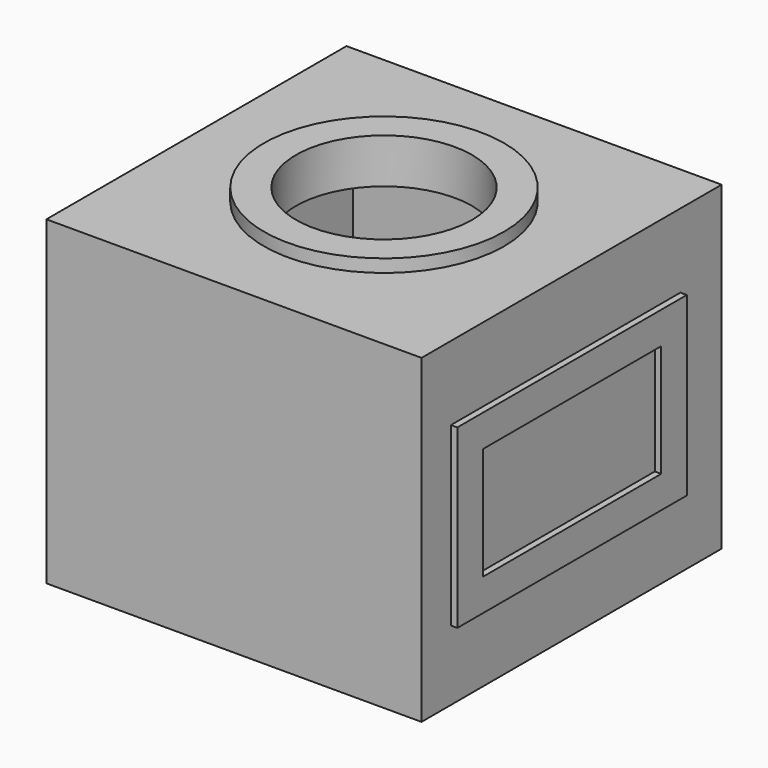
from build123d import *

# Parameters (mm, degrees)
F0_W          = 29.7304940177
F0_H          = 29.7304925771
F1_DEPTH      = 25.4
F2_R          = 9.516573444
F3_DEPTH      = 1.016
F4_T          = -2.54
F5_W          = 22.7350834757
F5_H          = 13.9908185229
F6_DEPTH      = 0.508
F7_T          = 2.54
F7_T3_DEPTH   = 25.4
F7_T5_DEPTH   = 29.7304925771
F7_T7_DEPTH   = 29.7304940177
F7_T9_DEPTH   = 27.8150834757
F7_T11_DEPTH  = 19.0708185229
F9_DEPTH      = 1.27
F10_T         = 2.54
F10_T3_DEPTH  = 25.4
F10_T5_DEPTH  = 29.7304925771
F10_T7_DEPTH  = 29.7304940177
F10_T9_DEPTH  = 20.819671886
F10_T11_DEPTH = 19.0130124822
F10_T13_DEPTH = 18.3381282199
F10_T15_DEPTH = 27.8150834757
F10_T17_DEPTH = 19.0708185229
F10_T19_DEPTH = 22.7350834757
F10_T21_DEPTH = 5.588
F10_T23_DEPTH = 13.9908185229
F12_DEPTH     = 1.016
F14_DEPTH     = 0.762


# Not quite as in the source:
# - a shell that OpenCascade refuses in one call is made with other operations: the cavity is built on its own and cut out


with BuildPart() as f1:
    # F0 (on Top) → F1 (new body)
    with BuildSketch(Plane.XY):
        with Locations((15.1567222201, 15.010983996)):
            Rectangle(F0_W, F0_H)
    extrude(amount=F1_DEPTH)

    # F2 (on face) → F3 (join)
    with BuildSketch(Plane.XY.offset(25.4)):
        with Locations((15.1567222201, 15.010983996)):
            Circle(F2_R)
    extrude(amount=F3_DEPTH)

    # F4
    f4_openings = [f1.faces().sort_by_distance(p)[0] for p in [
        (15.156722, 15.010984, 26.416),
    ]]
    offset(amount=F4_T, openings=f4_openings, kind=Kind.INTERSECTION)

    # F5 (on face) → F6 (join)
    with BuildSketch(Plane.YZ.offset(30.021969229)):
        with Locations((14.4280334935, 12.5334435143)):
            Rectangle(F5_W, F5_H)
    extrude(amount=F6_DEPTH)

    # F7: shell of thickness 2.54, made by hand


with BuildPart() as f7_core1:
    # F7_t2: copy of F1
    add(f1.part)

    # the walls: a layer under each face that stays
    f7_faces = [f7_core1.faces().sort_by_distance(p)[0] for p in [
        (2.8314752113, 15.010983996, 12.7),
        (15.1567222201, 27.3362302846, 12.7),
        (6.9398908809, 6.794153137, 22.86),
        (15.1567222201, 2.6857377075, 12.7),
        (15.1567222201, 15.010983996, 2.54),
        (27.481969229, 15.010983996, 12.7),
        (8.1801487762, 15.010983996, 24.638),
        (8.8123399241, 8.6666017001, 26.416),
        (5.6401487762, 15.010983996, 25.908),
        (5.2465575476, 5.1008198037, 25.4),
        (0.2914752113, 15.010983996, 12.7),
        (15.1567222201, 29.8762302846, 12.7),
        (15.1567222201, 0.1457377075, 12.7),
        (30.021969229, 5.1008198037, 21.1666666667),
        (15.1567222201, 15.010983996, 0),
        (30.275969229, 14.4280334935, 5.5380342528),
        (30.275969229, 3.0604917556, 12.5334435143),
        (30.275969229, 14.4280334935, 19.5288527757),
        (30.275969229, 25.7955752313, 12.5334435143),
    ]]
    thicken(f7_faces, amount=-F7_T, mode=Mode.SUBTRACT)

    # F7_s4 → F7_t3 (cut)
    with BuildSketch(Plane.XY):
        Polygon((2.8568752113, 27.3108302846), (0.2914752113, 27.3362302846), (0.2914752113, 29.8762302846), (2.8314752113, 29.8762302846), align=None)
        Polygon((2.8568752113, 2.7111377075), (0.2914752113, 2.6857377075), (0.2914752113, 0.1457377075), (2.8314752113, 0.1457377075), align=None)
        Polygon((27.456569229, 27.3108302846), (27.481969229, 29.8762302846), (30.021969229, 29.8762302846), (30.021969229, 27.3362302846), align=None)
        Polygon((27.456569229, 2.7111377075), (27.481969229, 0.1457377075), (30.021969229, 0.1457377075), (30.021969229, 2.6857377075), align=None)
    extrude(amount=F7_T3_DEPTH, mode=Mode.SUBTRACT)

    # F7_s6 → F7_t5 (cut)
    with BuildSketch(Plane.XZ.offset(-29.8762302846)):
        Polygon((2.8568752113, 22.8346), (0.2914752113, 22.86), (0.2914752113, 25.4), (2.8314752113, 25.4), align=None)
        Polygon((2.8568752113, 2.5654), (0.2914752113, 2.54), (0.2914752113, 0), (2.8314752113, 0), align=None)
        Polygon((27.456569229, 22.8346), (27.481969229, 25.4), (30.021969229, 25.4), (30.021969229, 22.86), align=None)
        Polygon((27.456569229, 2.5654), (27.481969229, 0), (30.021969229, 0), (30.021969229, 2.54), align=None)
    extrude(amount=F7_T5_DEPTH, mode=Mode.SUBTRACT)

    # F7_s8 → F7_t7 (cut)
    with BuildSketch(Plane.YZ.offset(0.2914752113)):
        Polygon((27.3108302846, 22.8346), (29.8762302846, 22.86), (29.8762302846, 25.4), (27.3362302846, 25.4), align=None)
        Polygon((27.3108302846, 2.5654), (29.8762302846, 2.54), (29.8762302846, 0), (27.3362302846, 0), align=None)
        Polygon((2.7111377075, 22.8346), (2.6857377075, 25.4), (0.1457377075, 25.4), (0.1457377075, 22.86), align=None)
        Polygon((2.7111377075, 2.5654), (0.1457377075, 2.54), (0.1457377075, 0), (2.6857377075, 0), align=None)
    extrude(amount=F7_T7_DEPTH, mode=Mode.SUBTRACT)

    # F7_s10 → F7_t9 (cut)
    with BuildSketch(Plane.XZ.offset(-28.3355752313)):
        Polygon((30.047369229, 5.5126342528), (27.481969229, 5.5380342528), (27.481969229, 8.0780342528), (30.021969229, 8.0780342528), align=None)
        Polygon((30.047369229, 19.5542527757), (27.481969229, 19.5288527757), (27.481969229, 16.9888527757), (30.021969229, 16.9888527757), align=None)
    extrude(amount=F7_T9_DEPTH, mode=Mode.SUBTRACT)

    # F7_s12 → F7_t11 (cut)
    with BuildSketch(Plane.XY.offset(2.9980342528)):
        Polygon((30.047369229, 3.0350917556), (27.481969229, 3.0604917556), (27.481969229, 5.6004917556), (30.021969229, 5.6004917556), align=None)
        Polygon((30.047369229, 25.8209752313), (27.481969229, 25.7955752313), (27.481969229, 23.2555752313), (30.021969229, 23.2555752313), align=None)
    extrude(amount=F7_T11_DEPTH, mode=Mode.SUBTRACT)

    # F7_s13 → F7_t14 (revolve, cut)
    with BuildSketch(Plane.XZ.offset(-15.010983996)):
        Polygon((24.6986956641, 25.4254), (22.1332956641, 25.4), (22.1332956641, 22.86), (24.6732956641, 22.86), align=None)
    revolve(axis=Axis((15.1567222201, 15.010983996, 25.4), (0, 0, 1)), mode=Mode.SUBTRACT)


with BuildPart() as f1_1:
    add(f1.part)

    # what is left inside the walls is the cavity
    f7_cavity = [f7_core1.part.solids().sort_by_distance(p)[0] for p in [
        (30.047369, 14.428033, 14.01858),
    ]]
    add(f7_cavity, mode=Mode.SUBTRACT)

    # F8 (on face) → F9 (join)
    with BuildSketch(Plane(origin=(0, 29.8762302846, 0), x_dir=(-1, 0, 0), z_dir=(0, 1, 0))):
        Polygon((-7.869835943, 8.3070490509), (-15.1567222201, 19.3831156939), (-23.609507829, 8.3070490509), (-15.1567222201, 8.3070490509), align=None)
    extrude(amount=F9_DEPTH)

    # F10: shell of thickness 2.54, made by hand


with BuildPart() as f10_core1:
    # F10_t2: copy of F1
    add(f1_1.part)

    # the walls: a layer under each face that stays
    f10_faces = [f10_core1.faces().sort_by_distance(p)[0] for p in [
        (2.8314752113, 15.010983996, 12.7),
        (15.1567222201, 27.3362302846, 12.7),
        (6.9398908809, 6.794153137, 22.86),
        (15.1567222201, 2.6857377075, 12.7),
        (15.1567222201, 15.010983996, 2.54),
        (27.481969229, 15.010983996, 12.7),
        (8.1801487762, 15.010983996, 24.638),
        (8.8123399241, 8.6666017001, 26.416),
        (5.6401487762, 15.010983996, 25.908),
        (5.2465575476, 5.1008198037, 25.4),
        (0.2914752113, 15.010983996, 12.7),
        (25.0668868927, 29.8762302846, 21.1666666667),
        (15.1567222201, 0.1457377075, 12.7),
        (30.021969229, 5.1008198037, 21.1666666667),
        (15.1567222201, 15.010983996, 0),
        (15.739671886, 30.5112302846, 8.3070490509),
        (19.3831150245, 30.5112302846, 13.8450823724),
        (11.5132790816, 30.5112302846, 13.8450823724),
        (30.275969229, 14.4280334935, 5.5380342528),
        (30.275969229, 3.0604917556, 12.5334435143),
        (30.275969229, 14.4280334935, 19.5288527757),
        (30.275969229, 25.7955752313, 12.5334435143),
        (30.529969229, 6.8496723349, 7.86983734),
        (30.275969229, 14.4280334935, 8.0780342528),
        (30.275969229, 23.2555752313, 12.5334435143),
        (30.275969229, 14.4280334935, 16.9888527757),
        (30.275969229, 5.6004917556, 12.5334435143),
        (30.021969229, 14.4280334935, 12.5334435143),
    ]]
    thicken(f10_faces, amount=-F10_T, mode=Mode.SUBTRACT)

    # F10_s4 → F10_t3 (cut)
    with BuildSketch(Plane.XY):
        Polygon((2.8568752113, 27.3108302846), (0.2914752113, 27.3362302846), (0.2914752113, 29.8762302846), (2.8314752113, 29.8762302846), align=None)
        Polygon((2.8568752113, 2.7111377075), (0.2914752113, 2.6857377075), (0.2914752113, 0.1457377075), (2.8314752113, 0.1457377075), align=None)
        Polygon((27.456569229, 27.3108302846), (27.481969229, 29.8762302846), (30.021969229, 29.8762302846), (30.021969229, 27.3362302846), align=None)
        Polygon((27.456569229, 2.7111377075), (27.481969229, 0.1457377075), (30.021969229, 0.1457377075), (30.021969229, 2.6857377075), align=None)
    extrude(amount=F10_T3_DEPTH, mode=Mode.SUBTRACT)

    # F10_s6 → F10_t5 (cut)
    with BuildSketch(Plane.XZ.offset(-29.8762302846)):
        Polygon((2.8568752113, 22.8346), (0.2914752113, 22.86), (0.2914752113, 25.4), (2.8314752113, 25.4), align=None)
        Polygon((2.8568752113, 2.5654), (0.2914752113, 2.54), (0.2914752113, 0), (2.8314752113, 0), align=None)
        Polygon((27.456569229, 22.8346), (27.481969229, 25.4), (30.021969229, 25.4), (30.021969229, 22.86), align=None)
        Polygon((27.456569229, 2.5654), (27.481969229, 0), (30.021969229, 0), (30.021969229, 2.54), align=None)
    extrude(amount=F10_T5_DEPTH, mode=Mode.SUBTRACT)

    # F10_s8 → F10_t7 (cut)
    with BuildSketch(Plane.YZ.offset(0.2914752113)):
        Polygon((27.3108302846, 22.8346), (29.8762302846, 22.86), (29.8762302846, 25.4), (27.3362302846, 25.4), align=None)
        Polygon((27.3108302846, 2.5654), (29.8762302846, 2.54), (29.8762302846, 0), (27.3362302846, 0), align=None)
        Polygon((2.7111377075, 22.8346), (2.6857377075, 25.4), (0.1457377075, 25.4), (0.1457377075, 22.86), align=None)
        Polygon((2.7111377075, 2.5654), (0.1457377075, 2.54), (0.1457377075, 0), (2.6857377075, 0), align=None)
    extrude(amount=F10_T7_DEPTH, mode=Mode.SUBTRACT)

    # F10_s10 → F10_t9 (cut)
    with BuildSketch(Plane.YZ.offset(5.329835943)):
        Polygon((29.9016302846, 8.2816490509), (27.3362302846, 8.3070490509), (27.3362302846, 10.8470490509), (29.8762302846, 10.8470490509), align=None)
    extrude(amount=F10_T9_DEPTH, mode=Mode.SUBTRACT)

    # F10_s12 → F10_t11 (cut)
    with BuildSketch(Plane(origin=(-5.3104872769, 0, 6.9585712577), x_dir=(0, 1, 0), z_dir=(0.6066732244, 0, -0.7949513185))):
        Polygon((29.9016302846, 23.8334736105), (27.3362302846, 23.8080736105), (27.3362302846, 21.2680736105), (29.8762302846, 21.2680736105), align=None)
    extrude(amount=F10_T11_DEPTH, mode=Mode.SUBTRACT)

    # F10_s14 → F10_t13 (cut)
    with BuildSketch(Plane(origin=(4.7955373639, 0, 7.2892164652), x_dir=(0, 1, 0), z_dir=(0.5496165187, 0, 0.8354170709))):
        Polygon((29.9016302846, -1.9835039116), (27.3362302846, -2.0089039116), (27.3362302846, -4.5489039116), (29.8762302846, -4.5489039116), align=None)
    extrude(amount=F10_T13_DEPTH, mode=Mode.SUBTRACT)

    # F10_s16 → F10_t15 (cut)
    with BuildSketch(Plane.XZ.offset(-28.3355752313)):
        Polygon((30.047369229, 5.5126342528), (27.481969229, 5.5380342528), (27.481969229, 8.0780342528), (30.021969229, 8.0780342528), align=None)
        Polygon((30.047369229, 19.5542527757), (27.481969229, 19.5288527757), (27.481969229, 16.9888527757), (30.021969229, 16.9888527757), align=None)
    extrude(amount=F10_T15_DEPTH, mode=Mode.SUBTRACT)

    # F10_s18 → F10_t17 (cut)
    with BuildSketch(Plane.XY.offset(2.9980342528)):
        Polygon((30.047369229, 3.0350917556), (27.481969229, 3.0604917556), (27.481969229, 5.6004917556), (30.021969229, 5.6004917556), align=None)
        Polygon((30.047369229, 25.8209752313), (27.481969229, 25.7955752313), (27.481969229, 23.2555752313), (30.021969229, 23.2555752313), align=None)
    extrude(amount=F10_T17_DEPTH, mode=Mode.SUBTRACT)

    # F10_s20 → F10_t19 (cut)
    with BuildSketch(Plane.XZ.offset(-25.7955752313)):
        Polygon((30.047369229, 8.1034342528), (30.021969229, 5.5380342528), (27.481969229, 5.5380342528), (27.481969229, 8.0780342528), align=None)
        Polygon((30.047369229, 16.9634527757), (30.021969229, 19.5288527757), (27.481969229, 19.5288527757), (27.481969229, 16.9888527757), align=None)
    extrude(amount=F10_T19_DEPTH, mode=Mode.SUBTRACT)

    # F10_s22 → F10_t21 (cut)
    with BuildSketch(Plane.YZ.offset(27.481969229)):
        Polygon((23.2301752313, 8.1034342528), (23.2555752313, 5.5380342528), (25.7955752313, 5.5380342528), (25.7955752313, 8.0780342528), align=None)
        Polygon((5.6258917556, 8.1034342528), (5.6004917556, 5.5380342528), (3.0604917556, 5.5380342528), (3.0604917556, 8.0780342528), align=None)
        Polygon((23.2301752313, 16.9634527757), (25.7955752313, 16.9888527757), (25.7955752313, 19.5288527757), (23.2555752313, 19.5288527757), align=None)
        Polygon((5.6258917556, 16.9634527757), (5.6004917556, 19.5288527757), (3.0604917556, 19.5288527757), (3.0604917556, 16.9888527757), align=None)
    extrude(amount=F10_T21_DEPTH, mode=Mode.SUBTRACT)

    # F10_s24 → F10_t23 (cut)
    with BuildSketch(Plane.XY.offset(5.5380342528)):
        Polygon((30.047369229, 23.2301752313), (30.021969229, 25.7955752313), (27.481969229, 25.7955752313), (27.481969229, 23.2555752313), align=None)
        Polygon((30.047369229, 5.6258917556), (30.021969229, 3.0604917556), (27.481969229, 3.0604917556), (27.481969229, 5.6004917556), align=None)
    extrude(amount=F10_T23_DEPTH, mode=Mode.SUBTRACT)

    # F10_s25 → F10_t26 (revolve, cut)
    with BuildSketch(Plane.XZ.offset(-15.010983996)):
        Polygon((24.6986956641, 25.4254), (22.1332956641, 25.4), (22.1332956641, 22.86), (24.6732956641, 22.86), align=None)
    revolve(axis=Axis((15.1567222201, 15.010983996, 25.4), (0, 0, 1)), mode=Mode.SUBTRACT)


with BuildPart() as f1_2:
    add(f1_1.part)

    # what is left inside the walls is the cavity
    f10_cavity = [f10_core1.part.solids().sort_by_distance(p)[0] for p in [
        (15.528605, 29.90163, 13.612435),
    ]]
    add(f10_cavity, mode=Mode.SUBTRACT)

    # F11 (on face) → F12 (join)
    with BuildSketch(Plane(origin=(0, 0, 0), x_dir=(1, 0, 0), z_dir=(0, 0, -1))):
        Polygon((25.0668860972, -7.4326233007), (11.6590168327, -7.4326233007), (5.8295079507, -24.3381969631), (18.0714763701, -24.3381969631), align=None)
    extrude(amount=F12_DEPTH)

    # F13 (on face) → F14 (join)
    with BuildSketch(Plane(origin=(0.2914752113, 0, 0), x_dir=(0, -1, 0), z_dir=(-1, 0, 0))):
        with BuildLine():
            add(Edge.make_bspline(
                [(-24.775410071, 20.5490160733), (-25.1740933695, 22.0975250298), (-4.6873757083, 23.1826141504), (-4.5267621045, 4.9664176824), (-27.8896118654, 3.6395127919), (-7.5312359208, 15.2818602681), (-24.4324130709, 19.2167959159), (-24.775410071, 20.5490160733)],
                knots=[0, 0, 0, 0, 0.2273070421, 0.4227963447, 0.6240019215, 0.804442188, 1, 1, 1, 1], degree=3))
        make_face()
    extrude(amount=F14_DEPTH)


solid = f1_2.part
